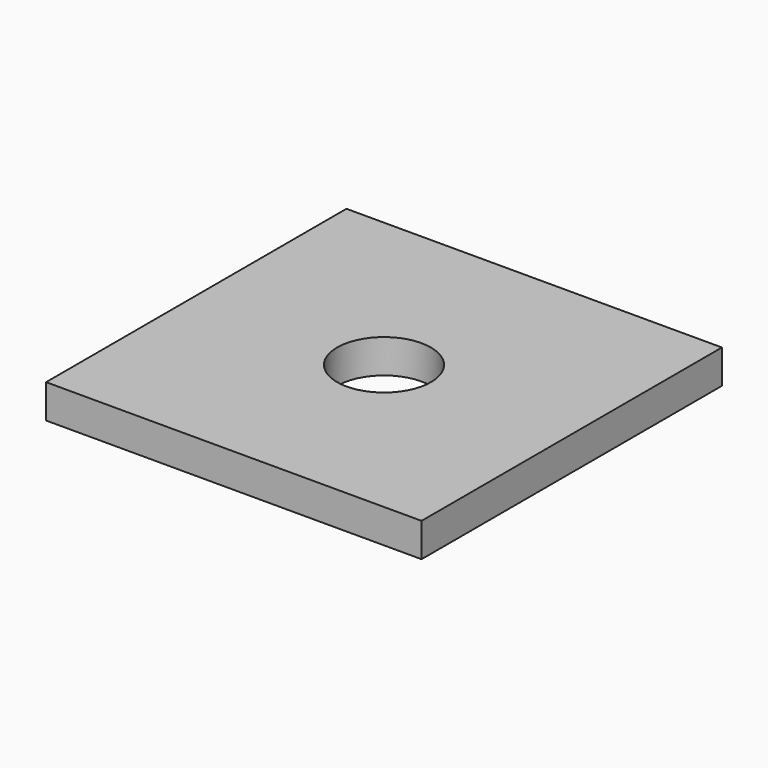
from build123d import *

# Parameters (mm, degrees)
F0_W     = 100
F0_H     = 100
F0_R     = 12.5
F1_DEPTH = 9


# Not quite as in the source:
# - a feature names something its author has since deleted; it is built from what else it names


with BuildPart() as f1:
    # F0 (on Top) → F1 (new body)
    with BuildSketch(Plane.XY):
        Rectangle(F0_W, F0_H)
        Circle(F0_R, mode=Mode.SUBTRACT)
    extrude(amount=F1_DEPTH)


solid = f1.part
